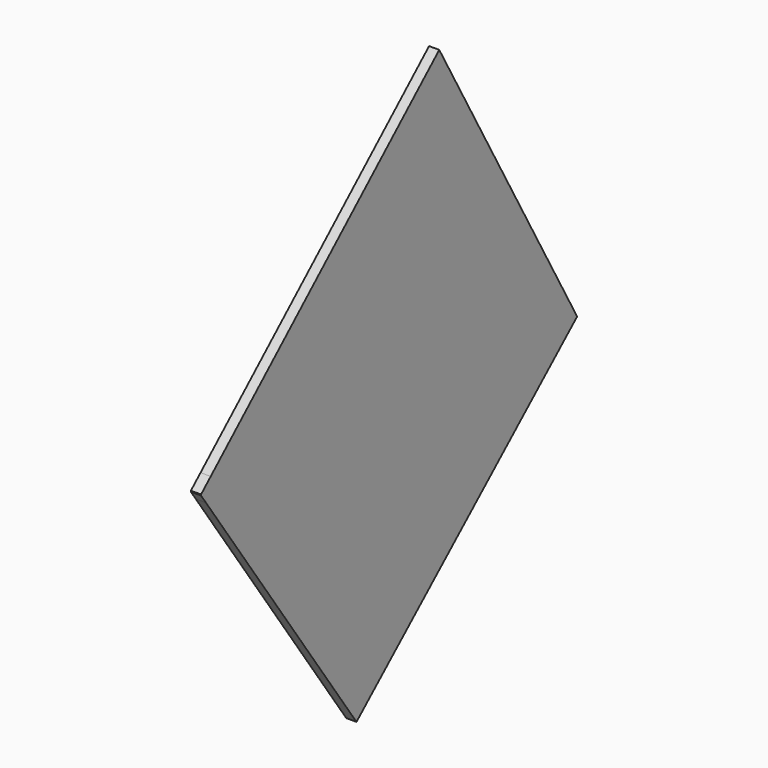
from build123d import *

# Parameters (mm, degrees)
F1_DEPTH = 1.3


with BuildPart() as f1:
    # F0 (on Right) → F1 (new body)
    with BuildSketch(Plane.YZ):
        with BuildLine():
            Line((-28.5022601296, 13.5822960047), (-30.0456807017, 12.1807558462))
            add(Edge.make_bspline(
                [(-30.0456807017, 12.1807558462), (-30.050324092, 12.1191925835), (-30.0456807017, 12.056948002)],
                knots=[0, 0, 0, 0.0248618931, 0.0248618931, 0.0248618931], degree=2, weights=[1, 0.9999227368, 1]))
            Line((-30.0456807017, 12.056948002), (-29.2544480902, 10.9238724842))
            add(Edge.make_bspline(
                [(-29.2544480902, 10.9238724842), (-6.4495956437, -6.866929483), (28.1840730012, 6.1202085385)],
                knots=[0.2427638345, 0.2427638345, 0.2427638345, 2.7999505323, 2.7999505323, 2.7999505323], degree=2, weights=[1, 0.2880625196, 1]))
            Line((28.1840730012, 6.1202085385), (30.0456807017, 7.7721911115))
            Line((30.0456807017, 7.7721911115), (29.5491017408, 8.6504284676))
            add(Edge.make_bspline(
                [(29.5491017408, 8.6504284676), (25.3237843176, 12.7552573017), (2.096655059, 14.7285637166), (-21.1304741996, 16.7018701315), (-28.5022601296, 13.5822960047)],
                knots=[3.3365042971, 3.3365042971, 3.3365042971, 4.6549863272, 4.6549863272, 5.9734683573, 5.9734683573, 5.9734683573], degree=2, weights=[1, 0.7904573504, 1, 0.7904573504, 1]))
        make_face()
        with BuildLine():
            Line((8.01217556, 46.7401072383), (-28.5022601296, 13.5822960047))
            add(Edge.make_bspline(
                [(29.5491017408, 8.6504284676), (25.3237843176, 12.7552573017), (2.096655059, 14.7285637166), (-21.1304741996, 16.7018701315), (-28.5022601296, 13.5822960047)],
                knots=[3.3365042971, 3.3365042971, 3.3365042971, 4.6549863272, 4.6549863272, 5.9734683573, 5.9734683573, 5.9734683573], degree=2, weights=[1, 0.7904573504, 1, 0.7904573504, 1]))
            Line((29.5491017408, 8.6504284676), (8.01217556, 46.7401072383))
        make_face()
        with BuildLine():
            add(Edge.make_bspline(
                [(-29.2544480902, 10.9238724842), (-6.4495956437, -6.866929483), (28.1840730012, 6.1202085385)],
                knots=[0.2427638345, 0.2427638345, 0.2427638345, 2.7999505323, 2.7999505323, 2.7999505323], degree=2, weights=[1, 0.2880625196, 1]))
            Line((-29.2544480902, 10.9238724842), (-5.2079111338, -23.5116928816))
            Line((-5.2079111338, -23.5116928816), (28.1840730012, 6.1202085385))
        make_face()
    extrude(amount=F1_DEPTH)


solid = f1.part
